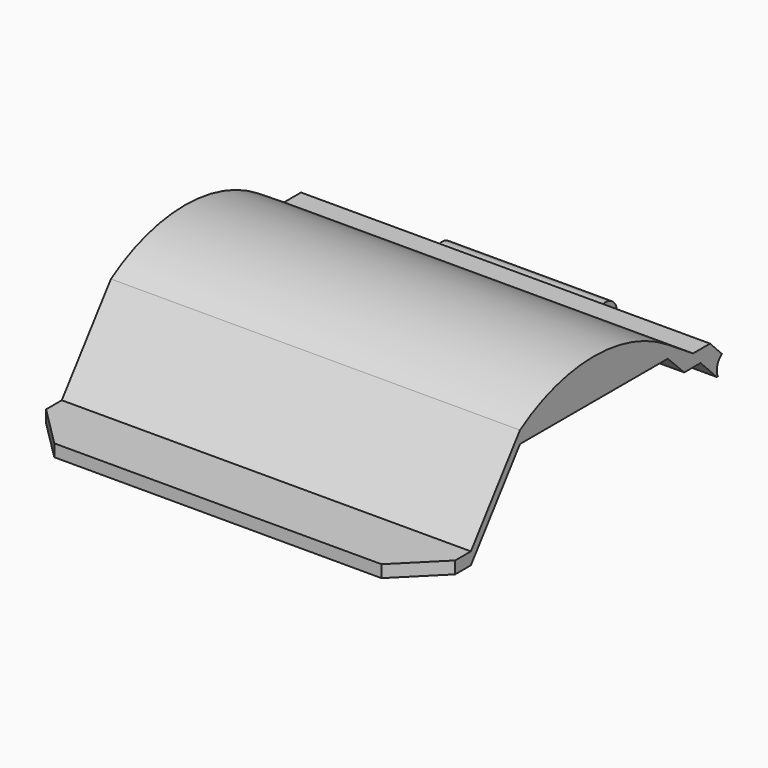
from build123d import *

# Parameters (mm, degrees)
F1_DEPTH  = 100
F2_SIZE   = 10
F3_R      = 3.5
F4_DEPTH  = 30
F5_R      = 3.6
F6_DEPTH  = 30
F7_R      = 1.125
F8_DEPTH  = 40
F11_DEPTH = 93


# Not quite as in the source:
# - a feature names something its author has since deleted; it is built from what else it names


with BuildPart() as f1:
    # F0 (on Right) → F1 (new body)
    with BuildSketch(Plane.YZ):
        with BuildLine():
            Line((25.5061486276, -1.4), (25.8561486276, -1.4))
            ThreePointArc((25.8561486276, -1.4), (32.4222243139, -0.9859028724), (27.1219938253, 2.9118378984))
            Line((27.1219938253, 2.9118378984), (23.5061486276, 6.6))
            Line((23.5061486276, 6.6), (18.2925903906, 6.6))
            Line((18.2925903906, 6.6), (10.6041878433, 11.6))
            Line((10.6041878433, 11.6), (-34.5898121567, 11.6))
            Line((-34.5898121567, 11.6), (-49.5898121567, -8.4))
            Line((-49.5898121567, -8.4), (-64.3958121567, -8.4))
            Line((-64.3958121567, -8.4), (-64.3958121567, -11.4))
            Line((-64.3958121567, -11.4), (-49.5898121567, -11.4))
            Line((-49.5898121567, -11.4), (-34.5898121567, 8.6))
            Line((-34.5898121567, 8.6), (10.6041878433, 8.6))
            Line((10.6041878433, 8.6), (15.6041878433, 3.6))
            Line((15.6041878433, 3.6), (20.6041878433, 3.6))
            Line((20.6041878433, 3.6), (25.5061486276, -1.4))
        make_face()
        with BuildLine():
            Line((-34.5898121567, 11.6), (10.6041878433, 11.6))
            ThreePointArc((10.6041878433, 11.6), (-11.9928121567, 18.3015086266), (-34.5898121567, 11.6))
        make_face()
    extrude(amount=F1_DEPTH)

    # F2
    f2_edges = [f1.edges().sort_by_distance(p)[0] for p in [
        (100, -64.395812, -9.9),
        (0, -64.395812, -9.9),
    ]]
    chamfer(f2_edges, length=F2_SIZE)

    # F3 (on face) → F4 (cut)
    with BuildSketch(Plane.YZ.offset(100)):
        with Locations((29.0639516141, 0)):
            Circle(F3_R)
    extrude(amount=-F4_DEPTH, mode=Mode.SUBTRACT)

    # F5 (on face) → F6 (cut)
    with BuildSketch(Plane(origin=(0, 0, 0), x_dir=(0, -1, 0), z_dir=(-1, 0, 0))):
        with Locations((-29.0639516141, 0)):
            Circle(F5_R)
    extrude(amount=-F6_DEPTH, mode=Mode.SUBTRACT)

    # F7 (on face) → F8 (cut, through all)
    with BuildSketch(Plane.YZ.offset(70)):
        with Locations((29.0639516141, 0)):
            Circle(F7_R)
    extrude(amount=-F8_DEPTH, mode=Mode.SUBTRACT)

    # F10 (on offset) → F11 (cut)
    with BuildSketch(Plane(origin=(3, 0, 0), x_dir=(0, -1, 0), z_dir=(-1, 0, 0))):
        with BuildLine():
            Line((-7.3898630986, 8.6), (31.992161455, 8.6))
            ThreePointArc((31.992161455, 8.6), (12.3011491782, 15.3028562463), (-7.3898630986, 8.6))
        make_face()
    extrude(amount=-F11_DEPTH, mode=Mode.SUBTRACT)


solid = f1.part
